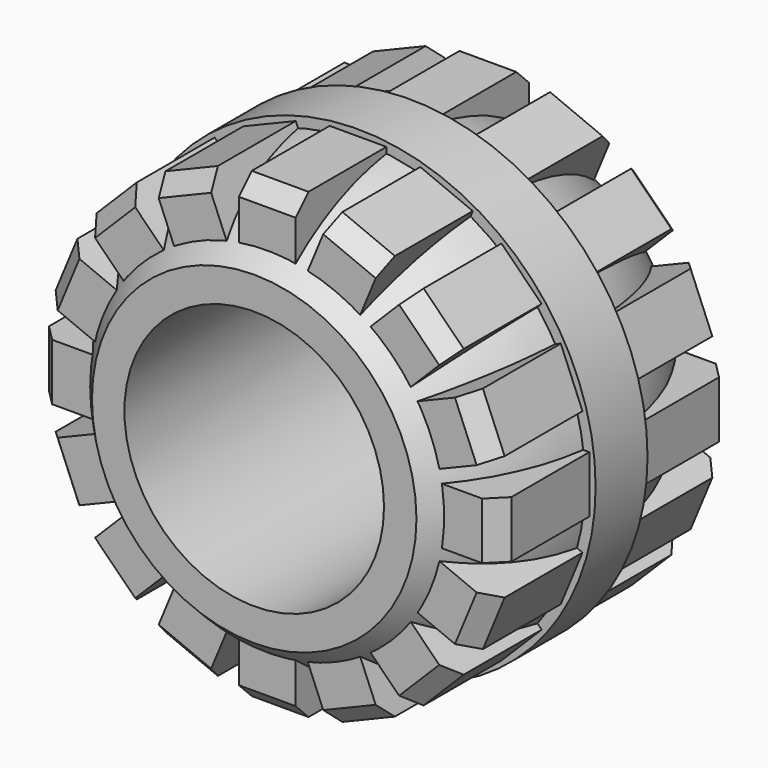
from build123d import *

# Parameters (mm, degrees)
F3_DEPTH = 180
F4_SIZE  = 20
F5_SIZE  = 20
F6_COUNT = 16


with BuildPart() as f1:
    # F0 (on Top) → F1 (revolve)
    with BuildSketch(Plane.XY):
        with BuildLine():
            Line((160, 200), (160, 0))
            Line((160, 0), (272.8427124746, 0))
            Line((272.8427124746, 0), (272.8427124746, 40))
            Line((272.8427124746, 40), (280, 40))
            ThreePointArc((280, 40), (252.9822128135, 126.4911064067), (200, 200))
            Line((200, 200), (160, 200))
        make_face()
        with BuildLine():
            Line((272.8427124746, 0), (160, 0))
            Line((160, 0), (160, -200))
            Line((160, -200), (200, -200))
            ThreePointArc((200, -200), (252.9822128135, -126.4911064067), (280, -40))
            Line((280, -40), (272.8427124746, -40))
            Line((272.8427124746, -40), (272.8427124746, 0))
        make_face()
    revolve(axis=Axis((0, 100, 0), (0, 1, 0)))


with BuildPart() as f1b:
    # F0 (on Top) → F1, piece 2 (revolve)
    with BuildSketch(Plane.XY):
        with BuildLine():
            ThreePointArc((280, 40), (282.1311392712, 20.0504427271), (282.8427124746, 0))
            ThreePointArc((282.8427124746, 0), (282.1311392712, -20.0504427271), (280, -40))
            Line((280, -40), (292.8427124746, -40))
            Line((292.8427124746, -40), (292.8427124746, 40))
            Line((292.8427124746, 40), (280, 40))
        make_face()
    revolve(axis=Axis((0, 100, 0), (0, 1, 0)))


with BuildPart() as f3:
    # F2 (on Front) → F3 (new body, symmetric)
    with BuildSketch(Plane.XZ):
        Polygon((35, 215), (35, 285), (-35, 285), (-35, 215), (0, 215), align=None)
    extrude(amount=F3_DEPTH, both=True)

    # F4
    f4_edges = [f3.edges().sort_by_distance(p)[0] for p in [
        (0, -180, 285),
    ]]
    chamfer(f4_edges, length=F4_SIZE)

    # F5
    f5_edges = [f3.edges().sort_by_distance(p)[0] for p in [
        (0, 180, 285),
    ]]
    chamfer(f5_edges, length=F5_SIZE)


with BuildPart() as f6_1:
    # F6: instance of F3
    add(f3.part.rotate(Axis((0, -40, 0), (0, 1, 0)), 1 * 360 / F6_COUNT))


with BuildPart() as f6_2:
    # F6: instance of F3
    add(f3.part.rotate(Axis((0, -40, 0), (0, 1, 0)), 2 * 360 / F6_COUNT))


with BuildPart() as f6_3:
    # F6: instance of F3
    add(f3.part.rotate(Axis((0, -40, 0), (0, 1, 0)), 3 * 360 / F6_COUNT))


with BuildPart() as f6_4:
    # F6: instance of F3
    add(f3.part.rotate(Axis((0, -40, 0), (0, 1, 0)), 4 * 360 / F6_COUNT))


with BuildPart() as f6_5:
    # F6: instance of F3
    add(f3.part.rotate(Axis((0, -40, 0), (0, 1, 0)), 5 * 360 / F6_COUNT))


with BuildPart() as f6_6:
    # F6: instance of F3
    add(f3.part.rotate(Axis((0, -40, 0), (0, 1, 0)), 6 * 360 / F6_COUNT))


with BuildPart() as f6_7:
    # F6: instance of F3
    add(f3.part.rotate(Axis((0, -40, 0), (0, 1, 0)), 7 * 360 / F6_COUNT))


with BuildPart() as f6_8:
    # F6: instance of F3
    add(f3.part.rotate(Axis((0, -40, 0), (0, 1, 0)), 8 * 360 / F6_COUNT))


with BuildPart() as f6_9:
    # F6: instance of F3
    add(f3.part.rotate(Axis((0, -40, 0), (0, 1, 0)), 9 * 360 / F6_COUNT))


with BuildPart() as f6_10:
    # F6: instance of F3
    add(f3.part.rotate(Axis((0, -40, 0), (0, 1, 0)), 10 * 360 / F6_COUNT))


with BuildPart() as f6_11:
    # F6: instance of F3
    add(f3.part.rotate(Axis((0, -40, 0), (0, 1, 0)), 11 * 360 / F6_COUNT))


with BuildPart() as f6_12:
    # F6: instance of F3
    add(f3.part.rotate(Axis((0, -40, 0), (0, 1, 0)), 12 * 360 / F6_COUNT))


with BuildPart() as f6_13:
    # F6: instance of F3
    add(f3.part.rotate(Axis((0, -40, 0), (0, 1, 0)), 13 * 360 / F6_COUNT))


with BuildPart() as f6_14:
    # F6: instance of F3
    add(f3.part.rotate(Axis((0, -40, 0), (0, 1, 0)), 14 * 360 / F6_COUNT))


with BuildPart() as f6_15:
    # F6: instance of F3
    add(f3.part.rotate(Axis((0, -40, 0), (0, 1, 0)), 15 * 360 / F6_COUNT))


solid = Compound([f1.part, f1b.part, f3.part, f6_1.part, f6_2.part, f6_3.part, f6_4.part, f6_5.part, f6_6.part, f6_7.part, f6_8.part, f6_9.part, f6_10.part, f6_11.part, f6_12.part, f6_13.part, f6_14.part, f6_15.part])
